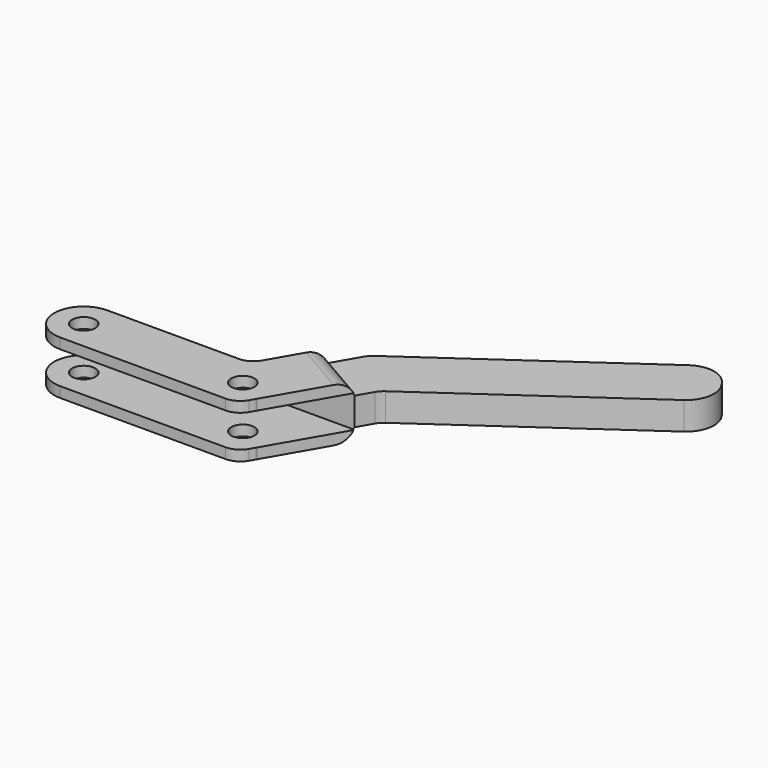
from build123d import *

# Parameters (mm, degrees)
F0_R          = 3.175
F1_DEPTH      = 3.81
F1_DEPTH_BACK = 3.81
F2_R          = 3.175
F3_DEPTH      = 3.4925
F3_DEPTH_BACK = 11.1125
F5_R          = 5.08
F6_R          = 7.62
F8_DEPTH      = 7.3025
F8_DEPTH_BACK = 7.3025
F4_W          = 35.6460946558
F4_H          = 8.89
F4_W_2        = 48.26
F4_W_3        = 30.9916705634
F9_DEPTH      = 23.5553863263
F10_T1_DEPTH  = 7.62
F10_T3_DEPTH  = 40.2569110938
F10_T5_DEPTH  = 13.2510444311
F10_T7_DEPTH  = 40.2569110938


# Not quite as in the source:
# - a fillet or chamfer that OpenCascade refuses, or shapes differently, is made with other operations: its cross-section is extruded or revolved along the edge and cut away or added


with BuildPart() as f1:
    # F0 (on Top) → F1 (new body, two sides)
    with BuildSketch(Plane.XY) as f1_sk:
        with BuildLine():
            Line((17.1451295545, 8.0645), (21.8027879538, 8.0645))
            ThreePointArc((21.8027879538, 8.0645), (28.7489728397, 4.0971545957), (28.860781215, -3.9013960801))
            Line((28.860781215, -3.9013960801), (42.9672120462, 20.531658833))
            Line((42.9672120462, 20.531658833), (102.5673909916, 62.2641534092))
            Line((102.5673909916, 62.2641534092), (93.2803106107, 75.5274787436))
            Line((93.2803106107, 75.5274787436), (30.8609248359, 31.8209542937))
            Line((30.8609248359, 31.8209542937), (17.1451295545, 8.0645))
        make_face()
        with BuildLine():
            ThreePointArc((28.7104927, -4.1617034239), (28.7868498226, -4.03225), (28.860781215, -3.9013960801))
            Line((28.860781215, -3.9013960801), (28.7104927, -4.1617034239))
        make_face()
        with BuildLine():
            ThreePointArc((28.860781215, -3.9013960801), (28.7489728397, 4.0971545957), (21.8027879538, 8.0645))
            Line((21.8027879538, 8.0645), (17.1451295545, 8.0645))
            Line((17.1451295545, 8.0645), (-21.8027879538, 8.0645))
            ThreePointArc((-21.8027879538, 8.0645), (-29.8672879538, 0), (-21.8027879538, -8.0645))
            Line((-21.8027879538, -8.0645), (21.8027879538, -8.0645))
            Line((21.8027879538, -8.0645), (26.4572120462, -8.0645))
            Line((26.4572120462, -8.0645), (28.7104927, -4.1617034239))
            Line((28.7104927, -4.1617034239), (28.860781215, -3.9013960801))
        make_face()
        with Locations((-21.8027879538, 0)):
            Circle(F0_R, mode=Mode.SUBTRACT)
        with Locations((21.8027879538, 0)):
            Circle(F0_R, mode=Mode.SUBTRACT)
    extrude(amount=F1_DEPTH)
    extrude(f1_sk.sketch, amount=-F1_DEPTH_BACK)

    # F2 (on face) → F3 (join, two sides)
    with BuildSketch(Plane.XY.offset(3.81)) as f3_sk:
        with BuildLine():
            Line((17.1451295545, 8.0645), (-21.8027879538, 8.0645))
            ThreePointArc((-21.8027879538, 8.0645), (-29.8672879538, 0), (-21.8027879538, -8.0645))
            Line((-21.8027879538, -8.0645), (26.4572120462, -8.0645))
            Line((26.4572120462, -8.0645), (28.7104927, -4.1617034239))
            ThreePointArc((28.7104927, -4.1617034239), (28.7868498226, -4.03225), (28.860781215, -3.9013960801))
            ThreePointArc((28.860781215, -3.9013960801), (28.7489728397, 4.0971545957), (21.8027879538, 8.0645))
            Line((21.8027879538, 8.0645), (17.1451295545, 8.0645))
        make_face()
        with Locations((-21.8027879538, 0)):
            Circle(F2_R, mode=Mode.SUBTRACT)
        with Locations((21.8027879538, 0)):
            Circle(F2_R, mode=Mode.SUBTRACT)
    extrude(amount=F3_DEPTH)
    extrude(f3_sk.sketch, amount=-F3_DEPTH_BACK)

    # F5
    f5_edges = [f1.edges().sort_by_distance(p)[0] for p in [
        (26.457212, -8.0645, 0),
        (17.14513, 8.0645, 0),
    ]]
    fillet(f5_edges, radius=F5_R)

    # F6
    f6_edges = [f1.edges().sort_by_distance(p)[0] for p in [
        (93.280311, 75.527479, 0),
        (102.567391, 62.264153, 0),
    ]]
    fillet(f6_edges, radius=F6_R)

    # F7 (on Top) → F8 (join, two sides)
    with BuildSketch(Plane.XY) as f8_sk:
        with BuildLine():
            Line((26.088796945, 23.5553863263), (18.6115992382, 10.6045))
            ThreePointArc((18.6115992382, 10.6045), (16.752190187, 8.7450909488), (14.212190187, 8.0645))
            Line((14.212190187, 8.0645), (21.8027879538, 8.0645))
            ThreePointArc((21.8027879538, 8.0645), (28.7489728397, 4.0971545957), (28.860781215, -3.9013960801))
            Line((28.860781215, -3.9013960801), (40.0569206826, 15.4908863263))
            Line((40.0569206826, 15.4908863263), (26.088796945, 23.5553863263))
        make_face()
    extrude(amount=F8_DEPTH)
    extrude(f8_sk.sketch, amount=-F8_DEPTH_BACK)

    # F4 (on face) → F9 (cut, through all)
    with BuildSketch(Plane.XZ.offset(8.0645)):
        with Locations((-39.6258352817, 0)):
            Rectangle(F4_W, F4_H)
        with Locations((2.3272120462, 0)):
            Rectangle(F4_W_2, F4_H)
        with Locations((41.9530473279, 0)):
            Rectangle(F4_W_3, F4_H)
    extrude(amount=-F9_DEPTH, mode=Mode.SUBTRACT)

    # F10: fillet of radius 5.08 on 4 edges, made by hand

    # F10_s2 → F10_t1 (join)
    with BuildSketch(Plane.XY.offset(-3.81)):
        with BuildLine():
            ThreePointArc((43.8897483577, 21.1776257125), (43.0581477833, 20.4483315822), (42.4041076031, 19.5563333275))
            Line((42.4041076031, 19.5563333275), (42.9672120462, 20.531658833))
            Line((42.9672120462, 20.531658833), (43.8897483577, 21.1776257125))
        make_face()
    extrude(amount=F10_T1_DEPTH)

    # F10_s4 → F10_t3 (cut)
    with BuildSketch(Plane(origin=(33.7826319428, -19.5044116461, 0), x_dir=(0, 0, 1), z_dir=(-0.8660254038, 0.5, 0))):
        with BuildLine():
            ThreePointArc((-3.81, 33.4439614271), (-6.3377703435, 31.5967932158), (-7.3025, 28.6183792083))
            Line((-7.3025, 28.6183792083), (-7.3025, 33.4439614271))
            Line((-7.3025, 33.4439614271), (-3.81, 33.4439614271))
        make_face()
    extrude(amount=F10_T3_DEPTH, mode=Mode.SUBTRACT)

    # F10_s6 → F10_t5 (cut)
    with BuildSketch(Plane.XY.offset(-6.6255222156)):
        with BuildLine():
            ThreePointArc((31.7834611474, 32.4669211732), (30.951860573, 31.7376270429), (30.2978203928, 30.8456287882))
            Line((30.2978203928, 30.8456287882), (30.8609248359, 31.8209542937))
            Line((30.8609248359, 31.8209542937), (31.7834611474, 32.4669211732))
        make_face()
    extrude(amount=F10_T5_DEPTH, mode=Mode.SUBTRACT)

    # F10_s8 → F10_t7 (cut)
    with BuildSketch(Plane(origin=(33.7826319428, -19.5044116461, 0), x_dir=(0, 0, 1), z_dir=(-0.8660254038, 0.5, 0))):
        with BuildLine():
            ThreePointArc((7.3025, 28.6183792083), (6.3377703435, 31.5967932158), (3.81, 33.4439614271))
            Line((3.81, 33.4439614271), (7.3025, 33.4439614271))
            Line((7.3025, 33.4439614271), (7.3025, 28.6183792083))
        make_face()
    extrude(amount=F10_T7_DEPTH, mode=Mode.SUBTRACT)


solid = f1.part
